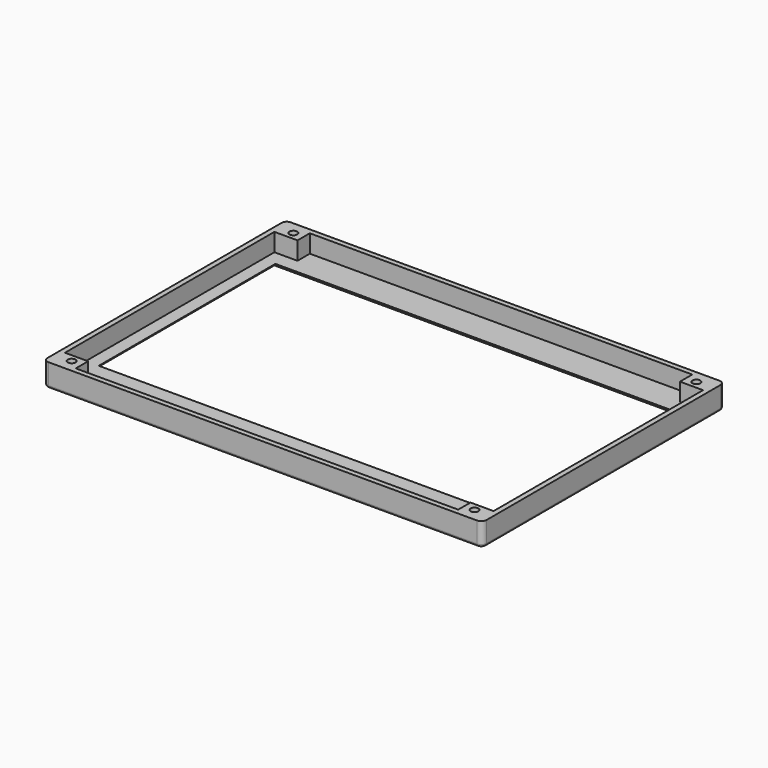
from build123d import *

# Parameters (mm, degrees)
F0_W          = 171
F0_H          = 118
F0_W_2        = 154
F0_H_2        = 86
F1_DEPTH      = 2
F2_SIZE       = 1.99999
F3_R          = 1
F4_W          = 171
F4_H          = 118
F4_W_2        = 167
F4_H_2        = 114
F5_DEPTH      = 7
F6_W          = 9
F6_H          = 6
F7_DEPTH      = 7
F8_R          = 1.525
F9_DEPTH      = 9.001
F10_T1_DEPTH  = 14
F10_T4_ANGLE  = 90
F10_T6_ANGLE  = 90
F10_T8_ANGLE  = 90
F10_T10_ANGLE = 90


# Not quite as in the source:
# - a fillet or chamfer that OpenCascade refuses, or shapes differently, is made with other operations: its cross-section is extruded or revolved along the edge and cut away or added
# - a fillet or chamfer is up to 0.001 mm smaller than in the source, because OpenCascade refuses the exact size


with BuildPart() as f1:
    # F0 (on Top) → F1 (new body)
    with BuildSketch(Plane.XY):
        with Locations((0.75, -1.11)):
            Rectangle(F0_W, F0_H)
        with Locations((-0.75, 1.11)):
            Rectangle(F0_W_2, F0_H_2, mode=Mode.SUBTRACT)
    extrude(amount=-F1_DEPTH)

    # F2 (size 2 in the source; OpenCascade refuses exactly that, so slightly less here)
    f2_edges = [f1.edges().sort_by_distance(p)[0] for p in [
        (76.25, 1.11, -2),
        (-0.75, -41.89, -2),
        (-0.75, 44.11, -2),
        (-77.75, 1.11, -2),
    ]]
    chamfer(f2_edges, length=F2_SIZE)

    # F3
    f3_edges = [f1.edges().sort_by_distance(p)[0] for p in [
        (-84.75, -1.11, -2),
        (0.75, -60.11, -2),
        (86.25, -1.11, -2),
        (0.75, 57.89, -2),
    ]]
    fillet(f3_edges, radius=F3_R)

    # F4 (on face) → F5 (join)
    with BuildSketch(Plane.XY):
        with Locations((0.75, -1.11)):
            Rectangle(F4_W, F4_H)
        with Locations((0.75, -1.11)):
            Rectangle(F4_W_2, F4_H_2, mode=Mode.SUBTRACT)
    extrude(amount=F5_DEPTH)

    # F6 (on face) → F7 (join)
    with BuildSketch(Plane.XY):
        with Locations((-78.25, 52.89)):
            Rectangle(F6_W, F6_H)
        with Locations((79.75, 52.89)):
            Rectangle(F6_W, F6_H)
        with Locations((79.75, -55.11)):
            Rectangle(F6_W, F6_H)
        with Locations((-78.25, -55.11)):
            Rectangle(F6_W, F6_H)
    extrude(amount=F7_DEPTH)

    # F8 (on face) → F9 (cut, through all)
    with BuildSketch(Plane(origin=(0, 0, -2), x_dir=(1, 0, 0), z_dir=(0, 0, -1))):
        with Locations((-77.75, 55.11)):
            Circle(F8_R)
        with Locations((79.25, 55.11)):
            Circle(F8_R)
        with Locations((-77.75, -52.89)):
            Circle(F8_R)
        with Locations((79.25, -52.89)):
            Circle(F8_R)
    extrude(amount=-F9_DEPTH, mode=Mode.SUBTRACT)

    # F10: fillet of radius 2 on 4 edges, made by hand

    # F10_s2 → F10_t1 (cut)
    with BuildSketch(Plane.XY.offset(-2)):
        with BuildLine():
            ThreePointArc((-84.75, 55.89), (-84.1642135624, 57.3042135624), (-82.75, 57.89))
            Line((-82.75, 57.89), (-84.75, 57.89))
            Line((-84.75, 57.89), (-84.75, 55.89))
        make_face()
        with BuildLine():
            ThreePointArc((84.25, 57.89), (85.6642135624, 57.3042135624), (86.25, 55.89))
            Line((86.25, 55.89), (86.25, 57.89))
            Line((86.25, 57.89), (84.25, 57.89))
        make_face()
        with BuildLine():
            ThreePointArc((84.25, -60.11), (85.6642135624, -59.5242135624), (86.25, -58.11))
            Line((86.25, -58.11), (86.25, -60.11))
            Line((86.25, -60.11), (84.25, -60.11))
        make_face()
        with BuildLine():
            ThreePointArc((-84.75, -58.11), (-84.1642135624, -59.5242135624), (-82.75, -60.11))
            Line((-82.75, -60.11), (-84.75, -60.11))
            Line((-84.75, -60.11), (-84.75, -58.11))
        make_face()
    extrude(amount=F10_T1_DEPTH, mode=Mode.SUBTRACT)

    # F10_s3 → F10_t4 (revolve, cut)
    with BuildSketch(Plane.YZ.offset(-82.75)):
        with BuildLine():
            ThreePointArc((-59.11, -2), (-59.8171067812, -1.7071067812), (-60.11, -1))
            Line((-60.11, -1), (-60.11, -2))
            Line((-60.11, -2), (-59.11, -2))
        make_face()
    revolve(axis=Axis((-82.75, -58.11, -2), (0, 0, -1)), revolution_arc=F10_T4_ANGLE, mode=Mode.SUBTRACT)

    # F10_s5 → F10_t6 (revolve, cut)
    with BuildSketch(Plane.XZ.offset(58.11)):
        with BuildLine():
            ThreePointArc((85.25, -2), (85.9571067812, -1.7071067812), (86.25, -1))
            Line((86.25, -1), (86.25, -2))
            Line((86.25, -2), (85.25, -2))
        make_face()
    revolve(axis=Axis((84.25, -58.11, -2), (0, 0, -1)), revolution_arc=F10_T6_ANGLE, mode=Mode.SUBTRACT)

    # F10_s7 → F10_t8 (revolve, cut)
    with BuildSketch(Plane.YZ.offset(84.25)):
        with BuildLine():
            ThreePointArc((56.89, -2), (57.5971067812, -1.7071067812), (57.89, -1))
            Line((57.89, -1), (57.89, -2))
            Line((57.89, -2), (56.89, -2))
        make_face()
    revolve(axis=Axis((84.25, 55.89, -2), (0, 0, -1)), revolution_arc=F10_T8_ANGLE, mode=Mode.SUBTRACT)

    # F10_s9 → F10_t10 (revolve, cut)
    with BuildSketch(Plane.XZ.offset(-55.89)):
        with BuildLine():
            ThreePointArc((-83.75, -2), (-84.4571067812, -1.7071067812), (-84.75, -1))
            Line((-84.75, -1), (-84.75, -2))
            Line((-84.75, -2), (-83.75, -2))
        make_face()
    revolve(axis=Axis((-82.75, 55.89, -2), (0, 0, -1)), revolution_arc=F10_T10_ANGLE, mode=Mode.SUBTRACT)


solid = f1.part
